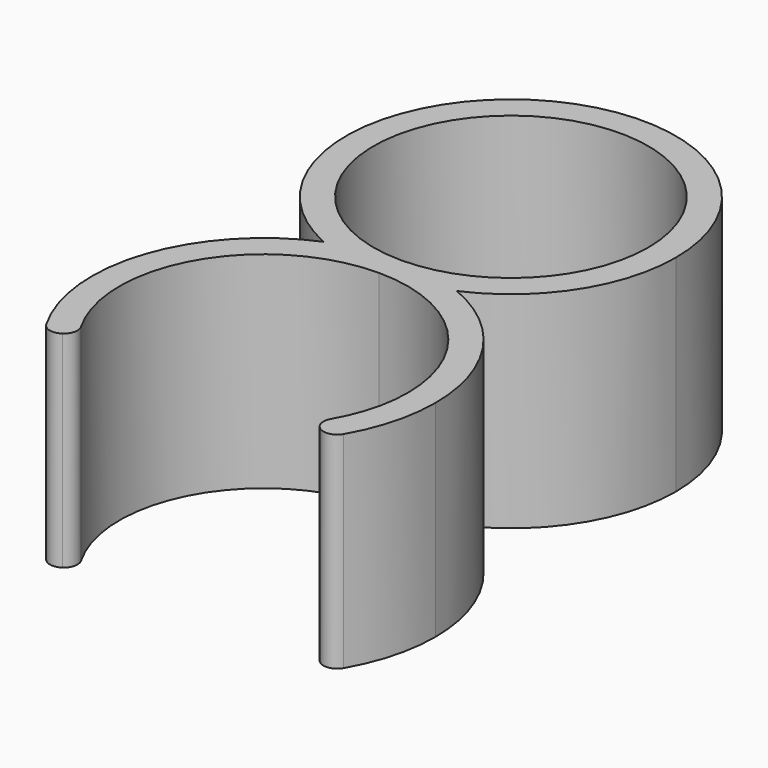
from build123d import *

# Parameters (mm, degrees)
F1_DEPTH = 15
F2_R     = 0.99999


# Not quite as in the source:
# - a fillet or chamfer is up to 0.001 mm smaller than in the source, because OpenCascade refuses the exact size


with BuildPart() as f1:
    # F0 (on Top) → F1 (new body)
    with BuildSketch(Plane.XY):
        with BuildLine():
            ThreePointArc((-4.8464827516, -10.9777777778), (-2.4720661624, -10.2468824829), (0, -10))
            ThreePointArc((0, -10), (2.4720661624, -10.2468824829), (4.8464827516, -10.9777777778))
            ThreePointArc((4.8464827516, -10.9777777778), (10.0538001029, -6.5514199598), (12, 0))
            ThreePointArc((12, 0), (-6.5514199598, 10.0538001029), (-4.8464827516, -10.9777777778))
        make_face()
        with BuildLine():
            ThreePointArc((0, -10), (-7.0710678119, 7.0710678119), (10, 0))
            ThreePointArc((10, 0), (7.0710678119, -7.0710678119), (0, -10))
        make_face(mode=Mode.SUBTRACT)
        with BuildLine():
            ThreePointArc((4.8464827516, -10.9777777778), (2.4720661624, -10.2468824829), (0, -10))
            ThreePointArc((0, -10), (-2.4720661624, -10.2468824829), (-4.8464827516, -10.9777777778))
            ThreePointArc((-4.8464827516, -10.9777777778), (-2.4765567495, -11.7416637095), (0, -12))
            ThreePointArc((0, -12), (2.4765567495, -11.7416637095), (4.8464827516, -10.9777777778))
        make_face()
        with BuildLine():
            ThreePointArc((12.5, -22.5), (10.412277234, -15.5837522599), (4.8464827516, -10.9777777778))
            ThreePointArc((4.8464827516, -10.9777777778), (2.4765567495, -11.7416637095), (0, -12))
            ThreePointArc((0, -12), (7.4246212025, -15.0753787975), (10.5, -22.5))
            ThreePointArc((10.5, -22.5), (10.0140279829, -25.6574108948), (8.601096465, -28.5225525817))
            Line((8.601096465, -28.5225525817), (10.2394005536, -29.6697054544))
            ThreePointArc((10.2394005536, -29.6697054544), (11.9214618844, -26.2588224938), (12.5, -22.5))
        make_face()
        with BuildLine():
            ThreePointArc((0, -12), (-2.4765567495, -11.7416637095), (-4.8464827516, -10.9777777778))
            ThreePointArc((-4.8464827516, -10.9777777778), (-12.0101211002, -19.034889445), (-10.2394005536, -29.6697054544))
            Line((-10.2394005536, -29.6697054544), (-8.601096465, -28.5225525817))
            ThreePointArc((-8.601096465, -28.5225525817), (-9.3136137484, -17.651639561), (0, -12))
        make_face()
    extrude(amount=F1_DEPTH)

    # F2 (radius 1 in the source; OpenCascade refuses exactly that, so slightly less here)
    f2_edges = [f1.edges().sort_by_distance(p)[0] for p in [
        (-8.601096, -28.522553, 7.5),
        (-10.239401, -29.669705, 7.5),
        (8.601096, -28.522553, 7.5),
        (10.239401, -29.669705, 7.5),
    ]]
    fillet(f2_edges, radius=F2_R)


solid = f1.part
